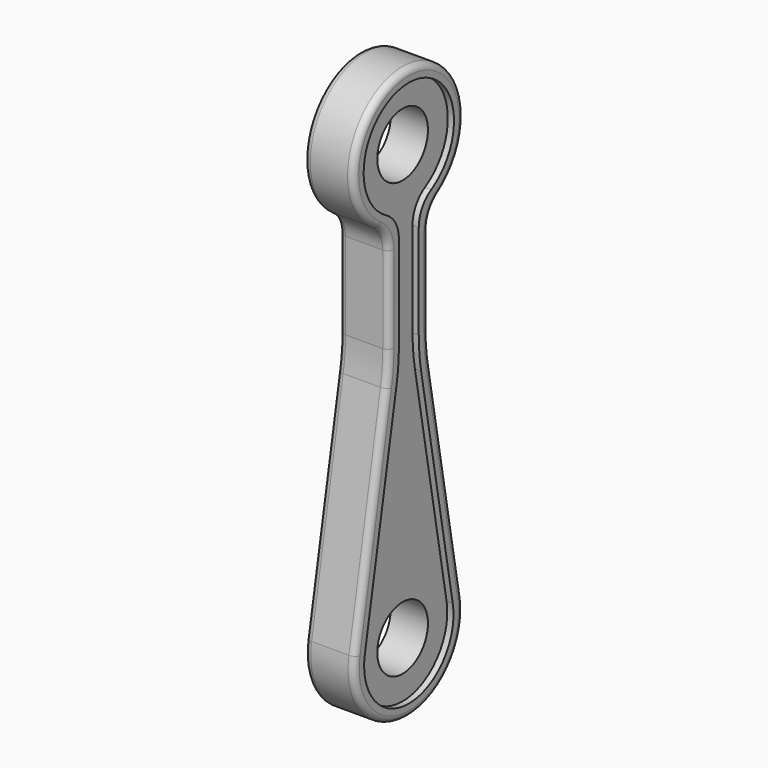
from build123d import *

# Parameters (mm, degrees)
F0_R     = 5.1
F1_DEPTH = 4
F2_R     = 5.1
F3_DEPTH = 1
F4_R     = 30
F5_R     = 5
F6_R     = 5
F7_R     = 30
F8_R     = 1
F9_R     = 1


# Not quite as in the source:
# - a pattern or mirror of a feature is missing from the dataset's text; its kind, count and spacing are read off the source's solid


with BuildPart() as f1:
    # F0 (on Right) → F1 (new body, symmetric)
    with BuildSketch(Plane.YZ):
        with BuildLine():
            ThreePointArc((4, -10.3542261903), (9.1545070867, -6.2773402011), (11.1, 0))
            ThreePointArc((11.1, 0), (-6.2773402011, 9.1545070867), (-4, -10.3542261903))
            ThreePointArc((-4, -10.3542261903), (0, -11.1), (4, -10.3542261903))
        make_face()
        Circle(F0_R, mode=Mode.SUBTRACT)
        with BuildLine():
            ThreePointArc((4, -10.3542261903), (0, -11.1), (-4, -10.3542261903))
            Line((-4, -10.3542261903), (-4, -30))
            Line((-4, -30), (-10.8271665456, -68.0577166546))
            ThreePointArc((-10.8271665456, -68.0577166546), (0, -59), (10.8271665456, -68.0577166546))
            Line((10.8271665456, -68.0577166546), (4, -30))
            Line((4, -30), (4, -10.3542261903))
        make_face()
        with BuildLine():
            ThreePointArc((10.8271665456, -68.0577166546), (0, -59), (-10.8271665456, -68.0577166546))
            ThreePointArc((-10.8271665456, -68.0577166546), (-0.9749789737, -80.9567064395), (11, -70))
            ThreePointArc((11, -70), (10.9567064395, -69.0250210263), (10.8271665456, -68.0577166546))
        make_face()
        with Locations((0, -70)):
            Circle(F0_R, mode=Mode.SUBTRACT)
    extrude(amount=F1_DEPTH, both=True)

    # F2 (on face) → F3 (cut)
    with BuildSketch(Plane.YZ.offset(4)):
        with BuildLine():
            Line((2, -30.1779693522), (2, -8.877499648))
            ThreePointArc((2, -8.877499648), (0, 9.1), (-2, -8.877499648))
            Line((-2, -8.877499648), (-2, -30.1779693522))
            Line((-2, -30.1779693522), (-8.85859081, -68.410859081))
            ThreePointArc((-8.85859081, -68.410859081), (0, -79), (8.85859081, -68.410859081))
            Line((8.85859081, -68.410859081), (2, -30.1779693522))
        make_face()
        with Locations((0, -70)):
            Circle(F2_R, mode=Mode.SUBTRACT)
        Circle(F2_R, mode=Mode.SUBTRACT)
    f3 = extrude(amount=-F3_DEPTH, mode=Mode.SUBTRACT)

    # F3_copies: F3 across plane
    add(f3.mirror(Plane(origin=(0, 0, 0), x_dir=(0, 0, -1), z_dir=(-1, 0, 0))), mode=Mode.SUBTRACT)

    # F4
    f4_edges = [f1.edges().sort_by_distance(p)[0] for p in [
        (0, -4, -30),
        (0, 4, -30),
    ]]
    fillet(f4_edges, radius=F4_R)

    # F5
    f5_edges = [f1.edges().sort_by_distance(p)[0] for p in [
        (0, -4, -10.354226),
        (0, 4, -10.354226),
    ]]
    fillet(f5_edges, radius=F5_R)

    # F6
    f6_edges = [f1.edges().sort_by_distance(p)[0] for p in [
        (3.5, -2, -8.8775),
        (3.5, 2, -8.8775),
        (-3.5, 2, -8.8775),
        (-3.5, -2, -8.8775),
    ]]
    fillet(f6_edges, radius=F6_R)

    # F7
    f7_edges = [f1.edges().sort_by_distance(p)[0] for p in [
        (-3.5, 2, -30.177969),
        (-3.5, -2, -30.177969),
        (3.5, 2, -30.177969),
        (3.5, -2, -30.177969),
    ]]
    fillet(f7_edges, radius=F7_R)

    # F8
    f8_edges = [f1.edges().sort_by_distance(p)[0] for p in [
        (4, 0, 11.1),
        (4, -4.585526, -11.001677),
        (4, -4, -20.339996),
        (4, -4.118073, -29.989493),
        (4, -7.649265, -50.342656),
        (4, 0, -81),
        (4, 7.649265, -50.342656),
        (4, 4.118073, -29.989493),
        (4, 4, -20.339996),
        (4, 4.585526, -11.001677),
    ]]
    fillet(f8_edges, radius=F8_R)

    # F9
    f9_edges = [f1.edges().sort_by_distance(p)[0] for p in [
        (-4, 0, 11.1),
        (-4, -4.585526, -11.001677),
        (-4, 4.585526, -11.001677),
        (-4, 4, -20.339996),
        (-4, -4, -20.339996),
        (-4, -4.118073, -29.989493),
        (-4, -7.649265, -50.342656),
        (-4, 0, -81),
        (-4, 7.649265, -50.342656),
        (-4, 4.118073, -29.989493),
    ]]
    fillet(f9_edges, radius=F9_R)


solid = f1.part
